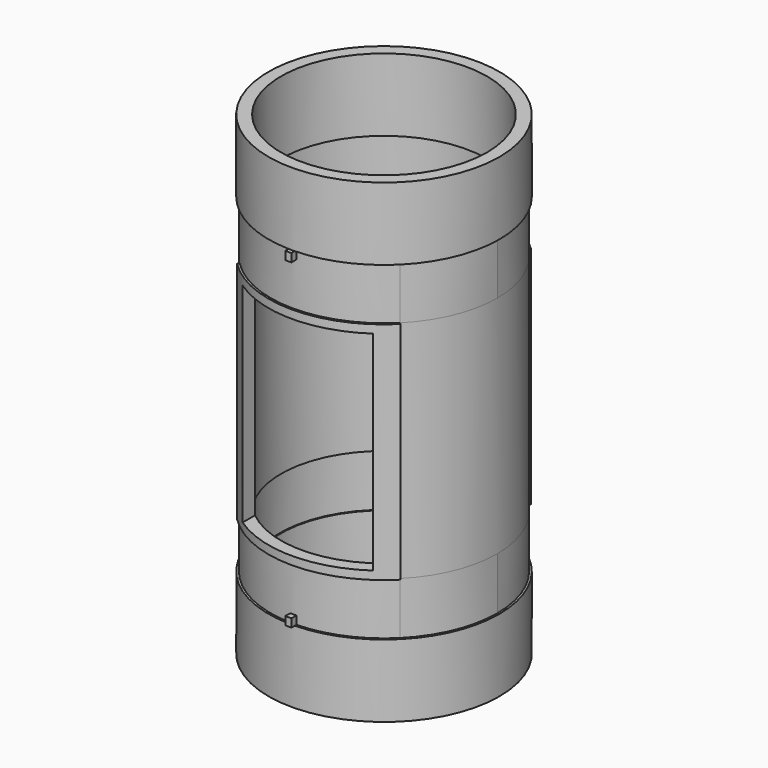
from build123d import *

# Parameters (mm, degrees)
F0_R           = 14
F1_DEPTH       = 57.6
F2_R           = 12.5
F3_DEPTH       = 57.601
F5_R           = 20.0664427739
F5_R_2         = 13.75
F6_DEPTH       = 6.35
F8_R           = 16.5527124134
F8_R_2         = 13.75
F9_DEPTH       = 6.35
F10_W          = 15.7989898732
F10_H          = 25.3
F11_DEPTH      = 14.001
F11_DEPTH_BACK = 25
F12_W          = 20.6221417799
F12_H          = 40
F13_ANGLE_BACK = 45
F13_ANGLE      = 90
F14_R          = 12.625
F15_DEPTH      = 6.35
F16_R          = 12.75
F17_DEPTH      = 6.35
F18_W          = 0.75
F18_H          = 1
F19_ANGLE_BACK = 1.5
F19_ANGLE      = 3


# Not quite as in the source:
# - after a boolean that leaves OpenCascade's solid faulty, fix() repairs it


with BuildPart() as f1:
    # F0 (on Top) → F1 (new body)
    with BuildSketch(Plane.XY):
        Circle(F0_R)
    extrude(amount=F1_DEPTH)

    # F2 (on face) → F3 (cut, through all)
    with BuildSketch(Plane.XY.offset(57.6)):
        Circle(F2_R)
    extrude(amount=-F3_DEPTH, mode=Mode.SUBTRACT)

    # F5 (on offset) → F6 (cut)
    with BuildSketch(Plane.XY.offset(8.8)):
        Circle(F5_R)
        Circle(F5_R_2, mode=Mode.SUBTRACT)
    extrude(amount=F6_DEPTH, mode=Mode.SUBTRACT)

    # F8 (on offset) → F9 (cut)
    with BuildSketch(Plane.XY.offset(48.8)):
        Circle(F8_R)
        Circle(F8_R_2, mode=Mode.SUBTRACT)
    extrude(amount=-F9_DEPTH, mode=Mode.SUBTRACT)

    # F10 (on Front) → F11 (cut, two sides)
    with BuildSketch(Plane.XZ) as f11_sk:
        with Locations((0, 28.8)):
            Rectangle(F10_W, F10_H)
    extrude(amount=F11_DEPTH, mode=Mode.SUBTRACT)
    extrude(f11_sk.sketch, amount=-F11_DEPTH_BACK, mode=Mode.SUBTRACT)

    # F12 (on Front) → F13 (revolve, cut)
    with BuildSketch(Plane.XZ, mode=Mode.PRIVATE) as f13_sk:
        with Locations((24.06107089, 28.8)):
            Rectangle(F12_W, F12_H)
        with Locations((-24.06107089, 28.8)):
            Rectangle(F12_W, F12_H)
    revolve(f13_sk.sketch.rotate(Axis((0, 0, 0), (0, 0, 1)), -F13_ANGLE_BACK), axis=Axis((0, 0, 0), (0, 0, 1)), revolution_arc=F13_ANGLE, mode=Mode.SUBTRACT)

    # F14 (on offset) → F15 (cut)
    with BuildSketch(Plane.XY.offset(8.8)):
        Circle(F14_R)
    extrude(amount=F15_DEPTH, mode=Mode.SUBTRACT)

    # F16 (on offset) → F17 (cut)
    with BuildSketch(Plane.XY.offset(48.8)):
        Circle(F16_R)
    extrude(amount=-F17_DEPTH, mode=Mode.SUBTRACT)

    # F18 (on Right) → F19 (revolve)
    with BuildSketch(Plane.YZ, mode=Mode.PRIVATE) as f19_sk:
        with Locations((-14.125, 48.3)):
            Rectangle(F18_W, F18_H)
        with Locations((14.125, 48.3)):
            Rectangle(F18_W, F18_H)
        with Locations((14.125, 9.3)):
            Rectangle(F18_W, F18_H)
        with Locations((-14.125, 9.3)):
            Rectangle(F18_W, F18_H)
    revolve(f19_sk.sketch.rotate(Axis((0, 0, 8.8), (0, 0, -1)), -F19_ANGLE_BACK), axis=Axis((0, 0, 8.8), (0, 0, -1)), revolution_arc=F19_ANGLE)

    add(f1.part.fix(), mode=Mode.REPLACE)


solid = f1.part
